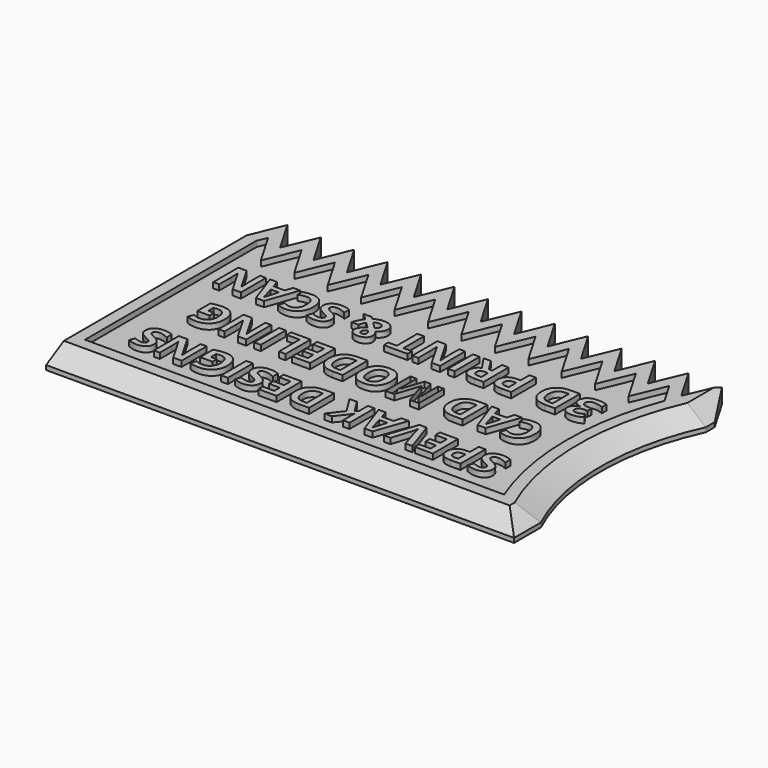
from build123d import *

# Parameters (mm, degrees)
F1_DEPTH     = 3
F2_SIZE2     = 4
F2_SIZE      = 2.2
F4_DEPTH     = 1
F5_TEXT_SIZE = 7.8708712652
F6_DEPTH     = 1


# Not quite as in the source:
# - Text() gives the source's letters only with a copy of the font that has no kerning and outlines rounded to 1/6400 em; it was checked with that copy


with BuildPart() as f1:
    # F0 (on Top) → F1 (new body)
    with BuildSketch(Plane.XY):
        with BuildLine():
            Line((0, 45), (0, 0))
            Line((0, 0), (84, 0))
            Line((84, 0), (84, 6))
            ThreePointArc((84, 6), (79.9290345012, 24.5), (84, 43))
            Line((84, 43), (84, 45))
            Line((84, 45), (80.5, 51))
            Line((80.5, 51), (78, 45))
            Line((78, 45), (74.5, 51))
            Line((74.5, 51), (72, 45))
            Line((72, 45), (68.5, 51))
            Line((68.5, 51), (66, 45))
            Line((66, 45), (62.5, 51))
            Line((62.5, 51), (60, 45))
            Line((60, 45), (56.5, 51))
            Line((56.5, 51), (54, 45))
            Line((54, 45), (50.5, 51))
            Line((50.5, 51), (48, 45))
            Line((48, 45), (44.5, 51))
            Line((44.5, 51), (42, 45))
            Line((42, 45), (38.5, 51))
            Line((38.5, 51), (36, 45))
            Line((36, 45), (32.5, 51))
            Line((32.5, 51), (30, 45))
            Line((30, 45), (26.5, 51))
            Line((26.5, 51), (24, 45))
            Line((24, 45), (20.5, 51))
            Line((20.5, 51), (18, 45))
            Line((18, 45), (14.5, 51))
            Line((14.5, 51), (12, 45))
            Line((12, 45), (8.5, 51))
            Line((8.5, 51), (6, 45))
            Line((6, 45), (2.5, 51))
            Line((2.5, 51), (0, 45))
        make_face()
    extrude(amount=F1_DEPTH)

    # F2
    f2_edges = [f1.edges().sort_by_distance(p)[0] for p in [
        (84, 44, 3),
        (79.929035, 24.5, 3),
        (42, 0, 3),
        (84, 3, 3),
    ]]
    chamfer(f2_edges, length=F2_SIZE, length2=F2_SIZE2)

    # F3 (on face) → F4 (cut)
    with BuildSketch(Plane.XY.offset(3)):
        with BuildLine():
            Line((2.8140926258, 46.2938223018), (2.1, 44.58))
            Line((2.1, 44.58), (2.1, 6.1))
            Line((2.1, 6.1), (77.3248912258, 6.1))
            ThreePointArc((77.3248912258, 6.1), (73.8298920243, 24.206666068), (77.1129278819, 42.3529618628))
            Line((77.1129278819, 42.3529618628), (74.8140926258, 46.2938223018))
            Line((74.8140926258, 46.2938223018), (72.3140926258, 40.2938223018))
            Line((72.3140926258, 40.2938223018), (68.8140926258, 46.2938223018))
            Line((68.8140926258, 46.2938223018), (66.3140926258, 40.2938223018))
            Line((66.3140926258, 40.2938223018), (62.8140926258, 46.2938223018))
            Line((62.8140926258, 46.2938223018), (60.3140926258, 40.2938223018))
            Line((60.3140926258, 40.2938223018), (56.8140926258, 46.2938223018))
            Line((56.8140926258, 46.2938223018), (54.3140926258, 40.2938223018))
            Line((54.3140926258, 40.2938223018), (50.8140926258, 46.2938223018))
            Line((50.8140926258, 46.2938223018), (48.3140926258, 40.2938223018))
            Line((48.3140926258, 40.2938223018), (44.8140926258, 46.2938223018))
            Line((44.8140926258, 46.2938223018), (42.3140926258, 40.2938223018))
            Line((42.3140926258, 40.2938223018), (38.8140926258, 46.2938223018))
            Line((38.8140926258, 46.2938223018), (36.3140926258, 40.2938223018))
            Line((36.3140926258, 40.2938223018), (32.8140926258, 46.2938223018))
            Line((32.8140926258, 46.2938223018), (30.3140926258, 40.2938223018))
            Line((30.3140926258, 40.2938223018), (26.8140926258, 46.2938223018))
            Line((26.8140926258, 46.2938223018), (24.3140926258, 40.2938223018))
            Line((24.3140926258, 40.2938223018), (20.8140926258, 46.2938223018))
            Line((20.8140926258, 46.2938223018), (18.3140926258, 40.2938223018))
            Line((18.3140926258, 40.2938223018), (14.8140926258, 46.2938223018))
            Line((14.8140926258, 46.2938223018), (12.3140926258, 40.2938223018))
            Line((12.3140926258, 40.2938223018), (8.8140926258, 46.2938223018))
            Line((8.8140926258, 46.2938223018), (6.3140926258, 40.2938223018))
            Line((6.3140926258, 40.2938223018), (2.8140926258, 46.2938223018))
        make_face()
    extrude(amount=-F4_DEPTH, mode=Mode.SUBTRACT)

    # F5 (on face) → F6 (join)
    with BuildSketch(Plane.XY.offset(2)):
        with Locations(Location((71.7395022511, 15.2025539428), (0, 0, -180))):
            Text('SPEVAK DESIGNS', F5_TEXT_SIZE, font='Open Sans', font_style=FontStyle.BOLD, text_align=(TextAlign.LEFT, TextAlign.BOTTOM))
        with Locations(Location((69.6943055458, 25.9069388635), (0, 0, -180))):
            Text('CAD MODELING', F5_TEXT_SIZE, font='Open Sans', font_style=FontStyle.BOLD, text_align=(TextAlign.LEFT, TextAlign.BOTTOM))
        with Locations(Location((71.7395022511, 36.6113237842), (0, 0, -180))):
            Text('3D PRINT & SCAN', F5_TEXT_SIZE, font='Open Sans', font_style=FontStyle.BOLD, text_align=(TextAlign.LEFT, TextAlign.BOTTOM))
    extrude(amount=F6_DEPTH)


solid = f1.part
